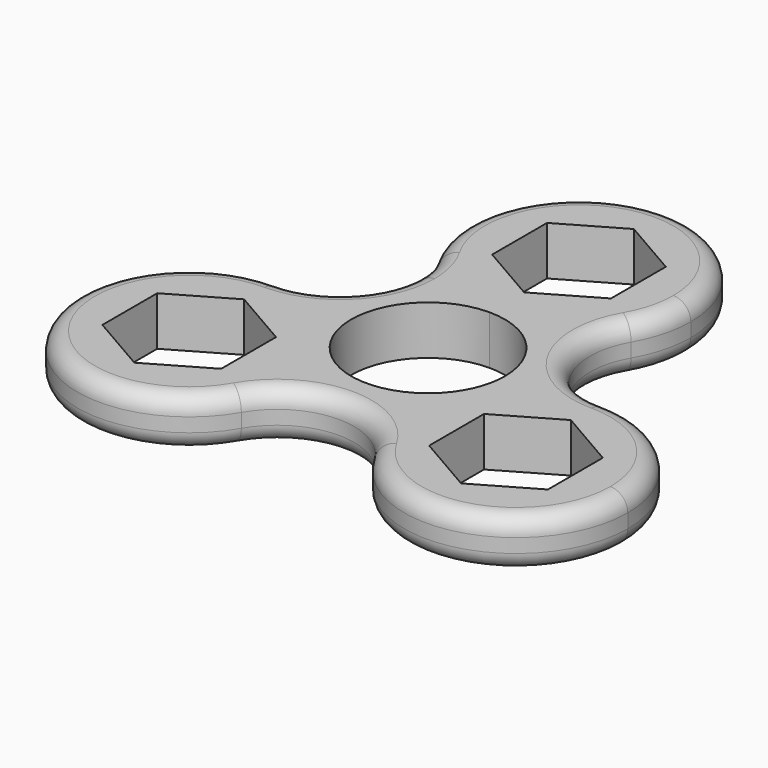
from build123d import *

# Parameters (mm, degrees)
F1_DEPTH = 7
F2_R     = 2.5


with BuildPart() as f1:
    # F0 (on Top) → F1 (new body)
    with BuildSketch(Plane.XY):
        with BuildLine():
            ThreePointArc((-9.5262794581, -5.4999999715), (-9.5262794251, 5.5000000286), (3.3e-08, 11))
            ThreePointArc((3.3e-08, 11), (-7.9999998612, 13.1435934593), (-13.8564063169, 18.9999997511))
            ThreePointArc((-13.8564063169, 18.9999997511), (-12.7575017758, 16.3470093573), (-12.3826859022, 13.5))
            ThreePointArc((-12.3826859022, 13.5), (-15.6045113091, 5.7218254069), (-23.3826859022, 2.5))
            ThreePointArc((-23.3826859022, 2.5), (-15.3826859164, 0.3564064688), (-9.5262794581, -5.4999999715))
        make_face()
        with BuildLine():
            ThreePointArc((-13.8564063169, 18.9999997511), (-7.9999998612, 13.1435934593), (3.3e-08, 11))
            ThreePointArc((3.3e-08, 11), (8.0000000671, 13.1435935782), (13.8564065215, 19.0000001056))
            ThreePointArc((13.8564065215, 19.0000001056), (15.4548132364, 22.8588953372), (16, 27))
            ThreePointArc((16, 27), (-4.1411048604, 42.4548131834), (-13.8564063169, 18.9999997511))
        make_face()
        Polygon((0, 36.8149545762), (8.5, 31.9074772881), (8.5, 22.0925227119), (0, 17.1850454238), (-8.5, 22.0925227119), (-8.5, 31.9074772881), align=None, mode=Mode.SUBTRACT)
        with BuildLine():
            ThreePointArc((3.3e-08, 11), (7.7781746047, 7.7781745814), (11, 0))
            ThreePointArc((11, 0), (10.6251840805, -2.8470095287), (9.5262794079, -5.5000000584))
            ThreePointArc((9.5262794079, -5.5000000584), (15.382685873, 0.3564064437), (23.3826859022, 2.5))
            ThreePointArc((23.3826859022, 2.5), (13.8564064301, 8.0000000528), (13.8564065215, 19.0000001056))
            ThreePointArc((13.8564065215, 19.0000001056), (8.0000000671, 13.1435935782), (3.3e-08, 11))
        make_face()
        with BuildLine():
            ThreePointArc((23.3826859022, 2.5), (15.382685873, 0.3564064437), (9.5262794079, -5.5000000584))
            ThreePointArc((9.5262794079, -5.5000000584), (7.3826859022, -13.5000000639), (9.5262794719, -21.5000000524))
            ThreePointArc((9.5262794719, -21.5000000524), (27.523790653, -28.9548132128), (39.3826859022, -13.5))
            ThreePointArc((39.3826859022, -13.5), (34.6963944012, -2.186291501), (23.3826859022, 2.5))
        make_face()
        Polygon((14.8826859022, -8.5925227119), (23.3826859022, -3.6850454238), (31.8826859022, -8.5925227119), (31.8826859022, -18.4074772881), (23.3826859022, -23.3149545762), (14.8826859022, -18.4074772881), align=None, mode=Mode.SUBTRACT)
        with BuildLine():
            ThreePointArc((9.5262794719, -21.5000000524), (7.3826859022, -13.5000000639), (9.5262794079, -5.5000000584))
            ThreePointArc((9.5262794079, -5.5000000584), (-5.02e-08, -11), (-9.5262794581, -5.4999999715))
            ThreePointArc((-9.5262794581, -5.4999999715), (-7.9278726858, -9.3588952624), (-7.3826859022, -13.5))
            ThreePointArc((-7.3826859022, -13.5), (-7.9278726602, -17.641104642), (-9.5262793592, -21.4999998571))
            ThreePointArc((-9.5262793592, -21.4999998571), (1.127e-07, -16), (9.5262794719, -21.5000000524))
        make_face()
        with BuildLine():
            ThreePointArc((-7.3826859022, -13.5), (-7.9278726858, -9.3588952624), (-9.5262794581, -5.4999999715))
            ThreePointArc((-9.5262794581, -5.4999999715), (-15.3826859164, 0.3564064688), (-23.3826859022, 2.5))
            ThreePointArc((-23.3826859022, 2.5), (-37.2390923215, -21.5000000714), (-9.5262793592, -21.4999998571))
            ThreePointArc((-9.5262793592, -21.4999998571), (-7.9278726602, -17.641104642), (-7.3826859022, -13.5))
        make_face()
        Polygon((-23.3826859022, -3.6850454238), (-14.8826859022, -8.5925227119), (-14.8826859022, -18.4074772881), (-23.3826859022, -23.3149545762), (-31.8826859022, -18.4074772881), (-31.8826859022, -8.5925227119), align=None, mode=Mode.SUBTRACT)
    extrude(amount=F1_DEPTH)

    # F2
    f2_edges = [f1.edges().sort_by_distance(p)[0] for p in [
        (0, 43, 7),
        (0, 43, 0),
        (13.856406, 8, 7),
        (13.856406, 8, 0),
        (37.239092, -21.5, 0),
        (37.239092, -21.5, 7),
        (0, -16, 7),
        (0, -16, 0),
        (-37.239092, -21.5, 0),
        (-37.239092, -21.5, 7),
        (-13.856407, 8, 7),
        (-13.856407, 8, 0),
    ]]
    fillet(f2_edges, radius=F2_R)


solid = f1.part
